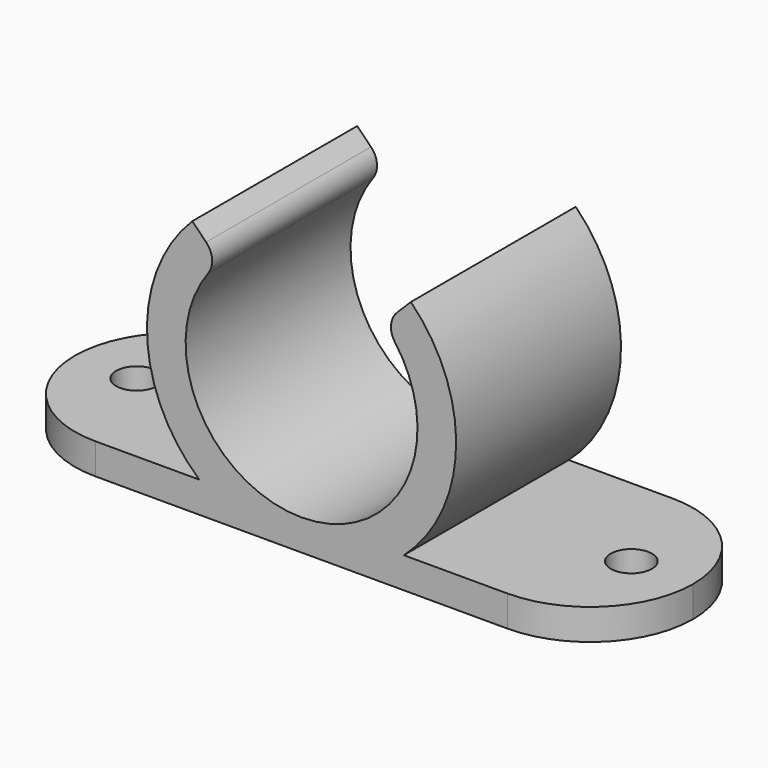
from build123d import *

# Parameters (mm, degrees)
F1_DEPTH = 20
F2_R     = 2
F3_R     = 2
F4_DEPTH = 25
F5_R     = 9.99999


# Not quite as in the source:
# - a fillet or chamfer is up to 0.001 mm smaller than in the source, because OpenCascade refuses the exact size


with BuildPart() as f1:
    # F0 (on Front) → F1 (new body)
    with BuildSketch(Plane.XZ):
        with BuildLine():
            Line((0, 3), (0, 0))
            Line((0, 0), (60, 0))
            Line((60, 0), (60, 3))
            Line((60, 3), (39.9215674165, 3))
            ThreePointArc((39.9215674165, 3), (44.9926379155, 13.7800975251), (40.6066017178, 24.8566017178))
            Line((40.6066017178, 24.8566017178), (37.9549512883, 22.2049512883))
            ThreePointArc((37.9549512883, 22.2049512883), (30, 3), (22.0450487117, 22.2049512883))
            Line((22.0450487117, 22.2049512883), (19.3933982822, 24.8566017178))
            ThreePointArc((19.3933982822, 24.8566017178), (15.0073620845, 13.7800975251), (20.0784325835, 3))
            Line((20.0784325835, 3), (0, 3))
        make_face()
    extrude(amount=F1_DEPTH)

    # F2
    f2_edges = [f1.edges().sort_by_distance(p)[0] for p in [
        (22.045049, -10, 22.204951),
        (37.954951, -10, 22.204951),
    ]]
    fillet(f2_edges, radius=F2_R)

    # F3 (on face) → F4 (cut)
    with BuildSketch(Plane.XY.offset(3)):
        with Locations((6, -10)):
            Circle(F3_R)
        with Locations((54, -10)):
            Circle(F3_R)
    extrude(amount=-F4_DEPTH, mode=Mode.SUBTRACT)

    # F5 (radius 10 in the source; OpenCascade refuses exactly that, so slightly less here)
    f5_edges = [f1.edges().sort_by_distance(p)[0] for p in [
        (0, 0, 1.5),
        (0, -20, 1.5),
        (60, -20, 1.5),
        (60, 0, 1.5),
    ]]
    fillet(f5_edges, radius=F5_R)


solid = f1.part
